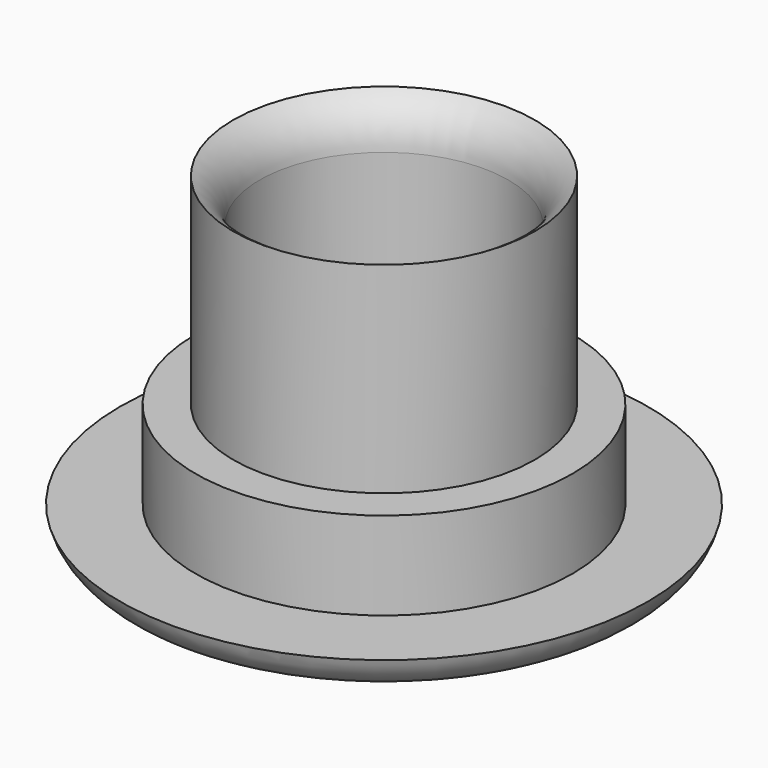
from build123d import *

# Parameters (mm, degrees)
F0_R     = 10.5
F0_R_2   = 7.5
F1_DEPTH = 1.5
F0_R_3   = 4.95
F2_DEPTH = 13
F4_R     = 7.5
F4_R_2   = 6
F5_DEPTH = 8


# Not quite as in the source:
# - a fillet or chamfer that OpenCascade refuses, or shapes differently, is made with other operations: its cross-section is extruded or revolved along the edge and cut away or added
# - a feature names something its author has since deleted; it is built from what else it names


with BuildPart() as f1:
    # F0 (on Top) → F1 (new body)
    with BuildSketch(Plane.XY):
        Circle(F0_R)
        Circle(F0_R_2, mode=Mode.SUBTRACT)
    extrude(amount=F1_DEPTH)

    # F0 (on Top) → F2 (join)
    with BuildSketch(Plane.XY):
        Circle(F0_R_2)
        Circle(F0_R_3, mode=Mode.SUBTRACT)
    extrude(amount=F2_DEPTH)

    # F3: fillet of radius 2 on 1 edges, made by hand

    # F3_s1 → F3_t2 (revolve, cut)
    with BuildSketch(Plane.XZ):
        with BuildLine():
            ThreePointArc((10.5, 1.5), (9.7882531983, 0.4188611699), (8.5635083269, 0))
            Line((8.5635083269, 0), (10.5, 0))
            Line((10.5, 0), (10.5, 1.5))
        make_face()
    revolve(axis=Axis((0, 0, 0), (0, 0, 1)), mode=Mode.SUBTRACT)

    # F4 (on face) → F5 (cut)
    with BuildSketch(Plane.XY.offset(13)):
        Circle(F4_R)
        Circle(F4_R_2, mode=Mode.SUBTRACT)
    extrude(amount=-F5_DEPTH, mode=Mode.SUBTRACT)

    # F6: fillet of radius 2 on 2 edges, made by hand

    # F6_s1 → F6_t2 (revolve, cut)
    with BuildSketch(Plane.XZ):
        with BuildLine():
            ThreePointArc((6.95, 0), (5.5357864376, 0.5857864376), (4.95, 2))
            Line((4.95, 2), (4.95, 0))
            Line((4.95, 0), (6.95, 0))
        make_face()
    revolve(axis=Axis((0, 0, 0), (0, 0, 1)), mode=Mode.SUBTRACT)

    # F6_s3 → F6_t4 (revolve, cut)
    with BuildSketch(Plane.XZ):
        with BuildLine():
            ThreePointArc((4.95, 11.2400284093), (5.2324435963, 12.2647234859), (6, 13))
            Line((6, 13), (4.95, 13))
            Line((4.95, 13), (4.95, 11.2400284093))
        make_face()
    revolve(axis=Axis((0, 0, 13), (0, 0, 1)), mode=Mode.SUBTRACT)


solid = f1.part
